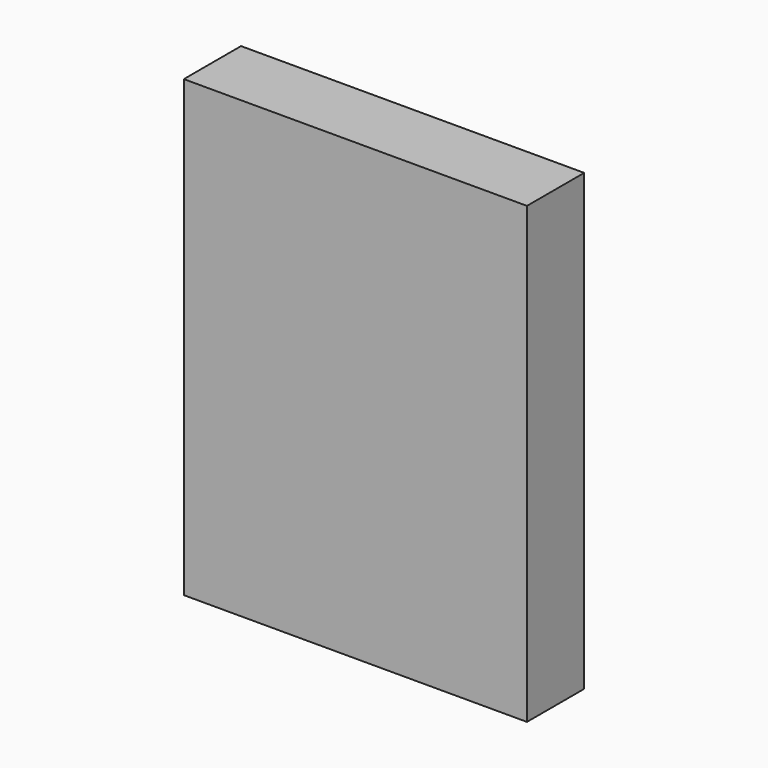
from build123d import *

# Parameters (mm, degrees)
F0_W          = 115.1676997542
F0_H          = 152.4667702615
F1_DEPTH      = 22
F1_DEPTH_BACK = 2


# Not quite as in the source:
# - the program builds the solid bodies; features that only make, move or delete a surface that nothing else refers to are left out


with BuildPart() as f1:
    # F0 (on Front) → F1 (new body, two sides)
    with BuildSketch(Plane.XZ) as f1_sk:
        with Locations((0, 0.0906009227)):
            Rectangle(F0_W, F0_H)
    extrude(amount=F1_DEPTH)
    extrude(f1_sk.sketch, amount=-F1_DEPTH_BACK)


solid = f1.part
